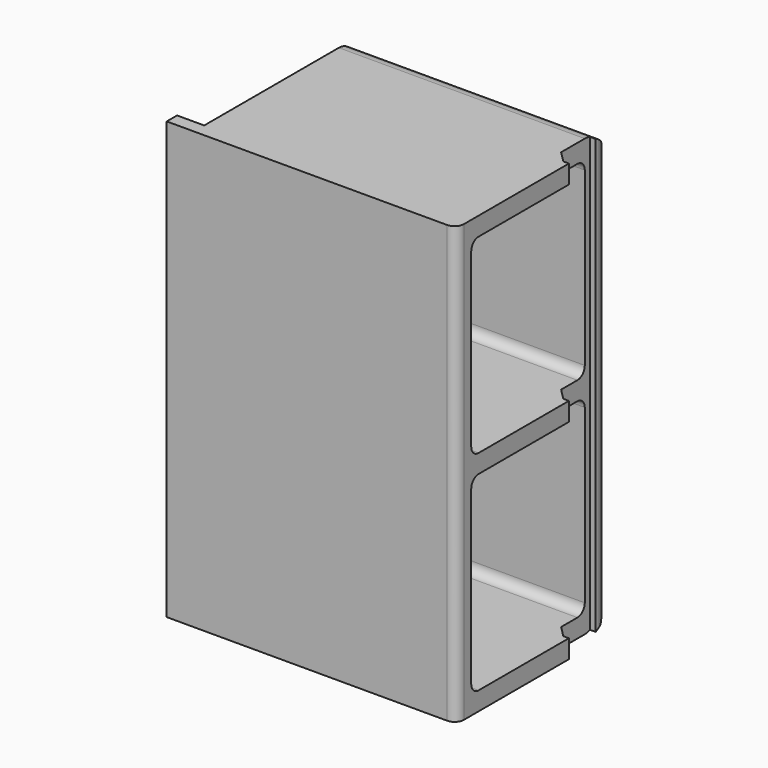
from build123d import *

# Parameters (mm, degrees)
F1_DEPTH    = 118
F4_DEPTH    = 61
F5_SIZE     = 2.49999
F6_R        = 5
F7_SIZE     = 3
F8_R        = 2.5
F9_T1_DEPTH = 118


# Not quite as in the source:
# - a fillet or chamfer that OpenCascade refuses, or shapes differently, is made with other operations: its cross-section is extruded or revolved along the edge and cut away or added
# - a fillet or chamfer is up to 0.001 mm smaller than in the source, because OpenCascade refuses the exact size


with BuildPart() as f1:
    # F0 (on Top) → F1 (new body)
    with BuildSketch(Plane.XY):
        Polygon((15.3875516164, 8.1571814393), (15.3875516164, 4.6571814393), (93.7208858402, 4.6571814393), (93.7208858402, 42.6571814393), (89.2208858402, 42.6571814393), (89.2208858402, 55.4571814393), (90.7208858402, 55.4571814393), (90.7208858402, 58.6571814393), (22.7208858402, 58.6571814393), (22.7208858402, 8.1571814393), align=None)
    extrude(amount=F1_DEPTH)

    # F3 (on face) → F4 (cut)
    with BuildSketch(Plane.YZ.offset(93.7208858402)):
        with BuildLine():
            Line((51.1571814393, 113), (42.6571814393, 113))
            Line((42.6571814393, 113), (42.6571814393, 61.5))
            Line((42.6571814393, 61.5), (51.1571814393, 61.5))
            ThreePointArc((51.1571814393, 61.5), (52.9249483923, 62.232233047), (53.6571814393, 64))
            Line((53.6571814393, 64), (53.6571814393, 110.5))
            ThreePointArc((53.6571814393, 110.5), (52.9249483923, 112.267766953), (51.1571814393, 113))
        make_face()
        with BuildLine():
            Line((42.6571814393, 61.5), (42.6571814393, 113))
            Line((42.6571814393, 113), (12.1571814393, 113))
            ThreePointArc((12.1571814393, 113), (10.3894144863, 112.267766953), (9.6571814393, 110.5))
            Line((9.6571814393, 110.5), (9.6571814393, 64))
            ThreePointArc((9.6571814393, 64), (10.3894144863, 62.232233047), (12.1571814393, 61.5))
            Line((12.1571814393, 61.5), (42.6571814393, 61.5))
        make_face()
        with BuildLine():
            Line((12.1571814393, 5), (42.6571814393, 5))
            Line((42.6571814393, 5), (42.6571814393, 56.5))
            Line((42.6571814393, 56.5), (12.1571814393, 56.5))
            ThreePointArc((12.1571814393, 56.5), (10.3894144863, 55.767766953), (9.6571814393, 54))
            Line((9.6571814393, 54), (9.6571814393, 7.5))
            ThreePointArc((9.6571814393, 7.5), (10.3894144863, 5.732233047), (12.1571814393, 5))
        make_face()
        with BuildLine():
            Line((42.6571814393, 56.5), (42.6571814393, 5))
            Line((42.6571814393, 5), (51.1571814393, 5))
            ThreePointArc((51.1571814393, 5), (52.9249483923, 5.732233047), (53.6571814393, 7.5))
            Line((53.6571814393, 7.5), (53.6571814393, 54))
            ThreePointArc((53.6571814393, 54), (52.9249483923, 55.767766953), (51.1571814393, 56.5))
            Line((51.1571814393, 56.5), (42.6571814393, 56.5))
        make_face()
    extrude(amount=-F4_DEPTH, mode=Mode.SUBTRACT)

    # F5 (size 2.5 in the source; OpenCascade refuses exactly that, so slightly less here)
    f5_edges = [f1.edges().sort_by_distance(p)[0] for p in [
        (32.720886, 52.924948, 112.267767),
        (32.720886, 31.657181, 113),
        (32.720886, 10.389414, 112.267767),
        (32.720886, 9.657181, 87.25),
        (32.720886, 10.389414, 62.232233),
        (32.720886, 31.657181, 61.5),
        (32.720886, 52.924948, 62.232233),
        (32.720886, 53.657181, 87.25),
        (32.720886, 10.389414, 5.732233),
        (32.720886, 31.657181, 5),
        (32.720886, 52.924948, 5.732233),
        (32.720886, 53.657181, 30.75),
        (32.720886, 52.924948, 55.767767),
        (32.720886, 31.657181, 56.5),
        (32.720886, 10.389414, 55.767767),
        (32.720886, 9.657181, 30.75),
    ]]
    chamfer(f5_edges, length=F5_SIZE)

    # F6
    f6_edges = [f1.edges().sort_by_distance(p)[0] for p in [
        (56.720886, 58.657181, 118),
        (56.720886, 58.657181, 0),
    ]]
    fillet(f6_edges, radius=F6_R)

    # F7
    f7_edges = [f1.edges().sort_by_distance(p)[0] for p in [
        (89.220886, 42.657181, 59),
        (89.220886, 42.657181, 2.5),
        (89.220886, 42.657181, 115.5),
    ]]
    chamfer(f7_edges, length=F7_SIZE)

    # F8
    f8_edges = [f1.edges().sort_by_distance(p)[0] for p in [
        (93.720886, 4.657181, 59),
    ]]
    fillet(f8_edges, radius=F8_R)

    # F9: fillet of radius 2 on 1 edges, made by hand

    # F9_s2 → F9_t1 (cut)
    with BuildSketch(Plane.XY):
        with BuildLine():
            ThreePointArc((90.7208858402, 56.6571814393), (90.1350994026, 58.0713950017), (88.7208858402, 58.6571814393))
            Line((88.7208858402, 58.6571814393), (90.7208858402, 58.6571814393))
            Line((90.7208858402, 58.6571814393), (90.7208858402, 56.6571814393))
        make_face()
    extrude(amount=F9_T1_DEPTH, mode=Mode.SUBTRACT)


solid = f1.part
